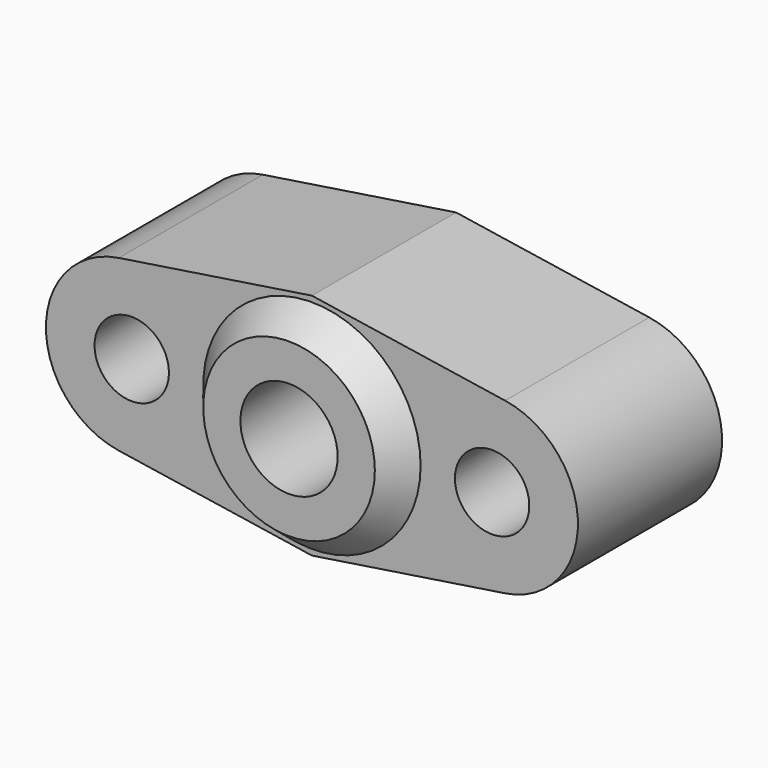
from build123d import *

# Parameters (mm, degrees)
F0_R      = 13
F0_R_2    = 38
F1_DEPTH  = 28
F3_R      = 30
F5_D      = 26
F6_D      = 26
F7_D      = 34
F7_DEPTH  = 28.001
F8_R      = 17
F9_DEPTH  = 25
F10_DEPTH = 35


# Not quite as in the source:
# - ends of sketch curves that miss each other by under 0.0002 mm in the source are joined


with BuildPart() as f1:
    # F0 (on Front) → F1 (new body)
    with BuildSketch(Plane.XZ):
        with BuildLine():
            Line((67.5423051658, 29.6541306361), (0, 40))
            Line((0, 40), (-67.5423051658, 29.6541306361))
            ThreePointArc((-67.5423051658, 29.6541306361), (-93, 0), (-67.5423051658, -29.6541306361))
            Line((-67.5423051658, -29.6541306361), (0, -40))
            Line((0, -40), (67.5423036859, -29.6541209752))
            ThreePointArc((67.5423036859, -29.6541209752), (67.5542752903, -29.6522946259), (67.5662446728, -29.6504537839))
            ThreePointArc((67.5662446728, -29.6504537839), (92.9999975558, 0.0121101119), (67.5423051658, 29.6541306361))
        make_face()
        with Locations((-63, 0)):
            Circle(F0_R, mode=Mode.SUBTRACT)
        Circle(F0_R_2, mode=Mode.SUBTRACT)
        with Locations((63, 0)):
            Circle(F0_R, mode=Mode.SUBTRACT)
        with Locations((-63, 0)):
            Circle(F0_R)
        Circle(F0_R_2)
        with Locations((63, 0)):
            Circle(F0_R)
    extrude(amount=-F1_DEPTH)

    # F3 (on offset) → F4 section 0
    with BuildSketch(Plane.XZ.offset(10)):
        Circle(F3_R)
    # F0 (on Front) → F4 section 1
    with BuildSketch(Plane.XZ):
        Circle(F0_R_2)
    loft()

    # F5 (through all)
    with Locations(Plane.XZ):
        with Locations((-63, 0)):
            Hole(F5_D / 2)

    # F6 (through all)
    with Locations(Plane.XZ):
        with Locations((63, 0)):
            Hole(F6_D / 2)

    # F7 (through all, one way)
    with BuildSketch(Plane.XZ):
        with Locations((0, 0)):
            Circle(F7_D / 2)
    extrude(amount=-F7_DEPTH, mode=Mode.SUBTRACT)

    # F8 (on face) → F9 (cut)
    with BuildSketch(Plane.XZ.offset(10)):
        Circle(F8_R)
    extrude(amount=-F9_DEPTH, mode=Mode.SUBTRACT)

    # F10 (add): a face of the model
    f10_faces = [f1.faces().sort_by_distance(p)[0] for p in [
        (90.975250823, 28, 0.0112927815),
    ]]
    extrude(f10_faces, amount=F10_DEPTH)


solid = f1.part
